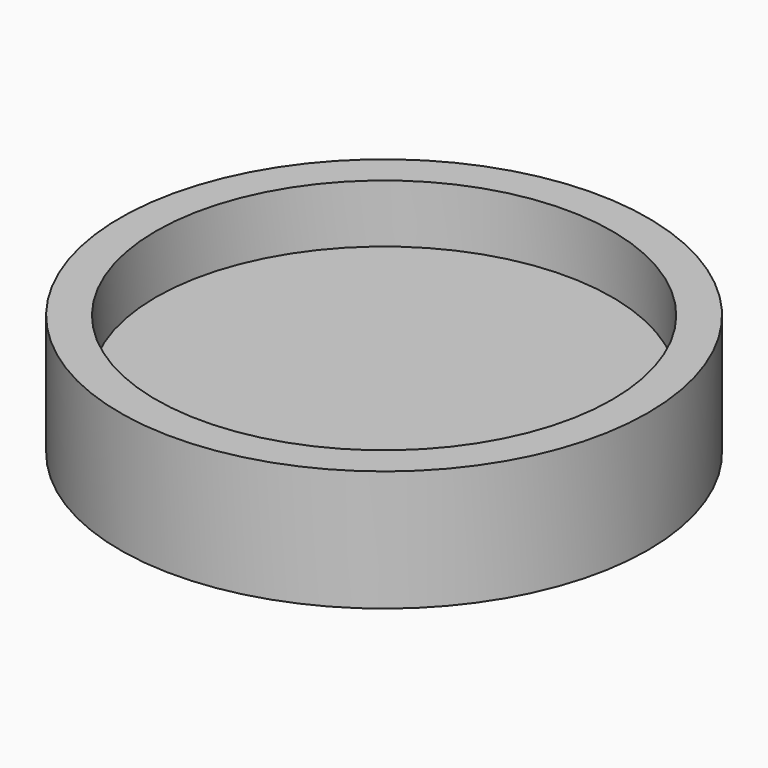
from build123d import *

# Parameters (mm, degrees)
F0_R     = 10
F1_DEPTH = 1
F2_R     = 11.8
F3_DEPTH = 1
F4_R     = 11.8
F4_R_2   = 10
F5_DEPTH = 1
F6_R     = 11.8
F7_DEPTH = 3.4
F8_R     = 10.2
F9_DEPTH = 2.6


with BuildPart() as f1:
    # F0 (on Top) → F1 (new body)
    with BuildSketch(Plane.XY):
        Circle(F0_R)
    extrude(amount=F1_DEPTH)


with BuildPart() as f3:
    # F2 (on face) → F3 (new body)
    with BuildSketch(Plane(origin=(0, 0, 0), x_dir=(1, 0, 0), z_dir=(0, 0, -1))):
        Circle(F2_R)
    extrude(amount=F3_DEPTH)

    # F4 (on face) → F5 (join)
    with BuildSketch(Plane.XY):
        Circle(F4_R)
        Circle(F4_R_2, mode=Mode.SUBTRACT)
    extrude(amount=F5_DEPTH)

    # F6 (on face) → F7 (join)
    with BuildSketch(Plane.XY.offset(1)):
        Circle(F6_R)
    extrude(amount=F7_DEPTH)

    # F8 (on face) → F9 (cut)
    with BuildSketch(Plane.XY.offset(4.4)):
        Circle(F8_R)
    extrude(amount=-F9_DEPTH, mode=Mode.SUBTRACT)


solid = Compound([f1.part, f3.part])
